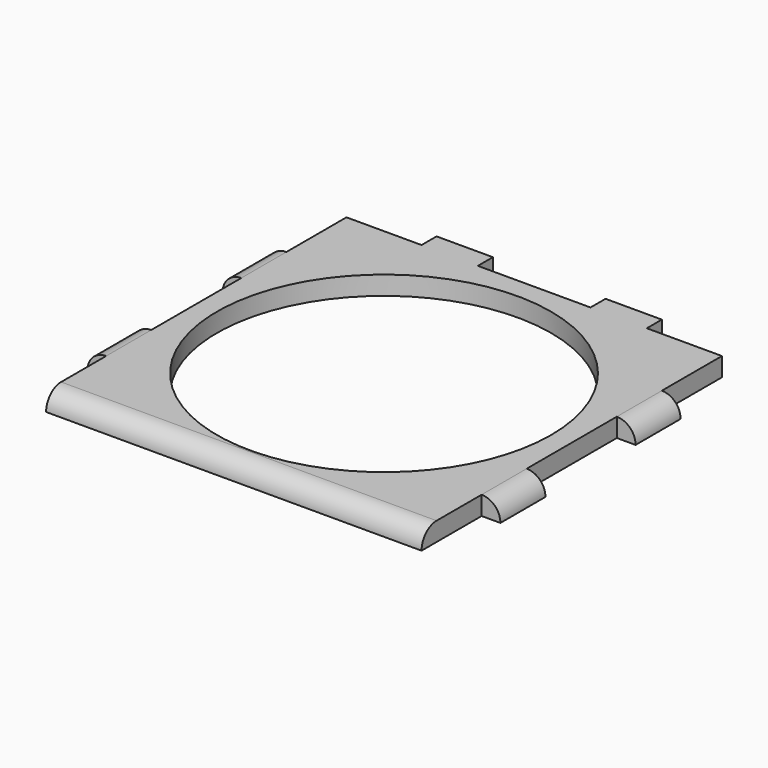
from build123d import *

# Parameters (mm, degrees)
F0_R     = 44.5
F1_DEPTH = 5
F2_R     = 4.99999


# Not quite as in the source:
# - a fillet or chamfer is up to 0.001 mm smaller than in the source, because OpenCascade refuses the exact size


with BuildPart() as f1:
    # F0 (on Top) → F1 (new body)
    with BuildSketch(Plane.XY):
        Polygon((-30, 50), (-50, 50), (-50, 30), (-55, 30), (-55, 15), (-50, 15), (-50, -15), (-55, -15), (-55, -30), (-50, -30), (-50, -50), (50, -50), (50, -30), (55, -30), (55, -15), (50, -15), (50, 15), (55, 15), (55, 30), (50, 30), (50, 50), (30, 50), (30, 55), (15, 55), (15, 50), (-15, 50), (-15, 55), (-30, 55), align=None)
        Circle(F0_R, mode=Mode.SUBTRACT)
    extrude(amount=F1_DEPTH)

    # F2 (radius 5 in the source; OpenCascade refuses exactly that, so slightly less here)
    f2_edges = [f1.edges().sort_by_distance(p)[0] for p in [
        (0, -50, 5),
        (55, -22.5, 5),
        (55, 22.5, 5),
        (-55, 22.5, 5),
        (-55, -22.5, 5),
    ]]
    fillet(f2_edges, radius=F2_R)


solid = f1.part
